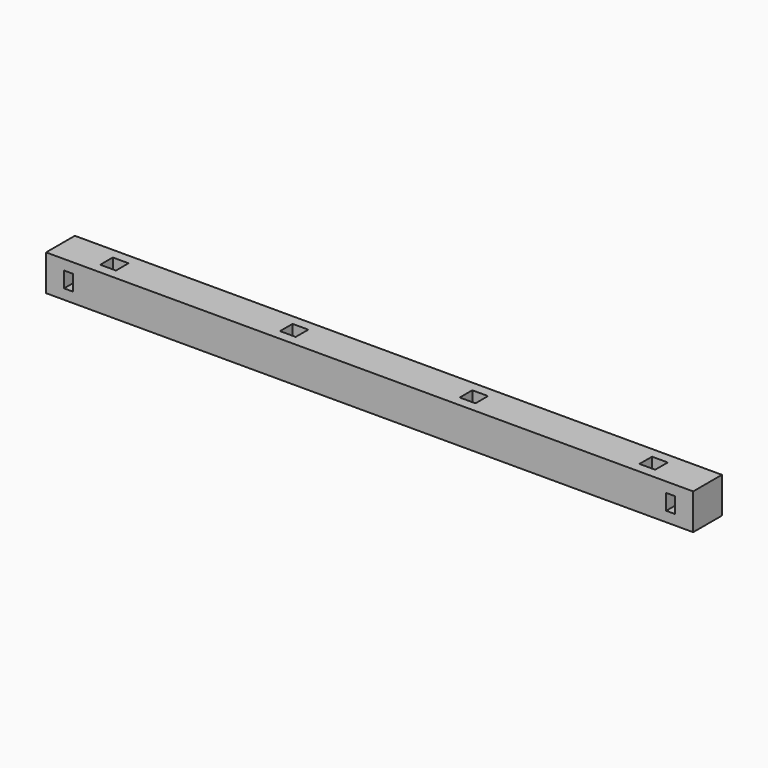
from build123d import *

# Parameters (mm, degrees)
F0_W            = 101.6
F0_H            = 101.6
F1_DEPTH        = 914.4
F2_W            = 44.45
F2_H            = 44.45
F3_DEPTH        = 101.601
F4_W            = 44.45
F4_H            = 44.45
F5_DEPTH        = 101.601
F5_COPIES_COUNT = 3
F5_COPIES_PITCH = 508
F6_W            = 25.4
F6_H            = 44.45
F7_DEPTH        = 101.601


# Not quite as in the source:
# - a pattern or mirror of a feature is missing from the dataset's text; its kind, count and spacing are read off the source's solid


with BuildPart() as f1:
    # F0 (on Right) → F1 (new body, symmetric)
    with BuildSketch(Plane.YZ):
        Rectangle(F0_W, F0_H)
    extrude(amount=F1_DEPTH, both=True)

    # F2 (on face) → F3 (cut, through all)
    with BuildSketch(Plane.XY.offset(50.8)):
        with Locations((-762, 0)):
            Rectangle(F2_W, F2_H)
    extrude(amount=-F3_DEPTH, mode=Mode.SUBTRACT)

    # F4 (on face) → F5 (cut, through all)
    with BuildSketch(Plane.XY.offset(50.8)):
        with Locations((-254, 0)):
            Rectangle(F4_W, F4_H)
    f5 = extrude(amount=-F5_DEPTH, mode=Mode.SUBTRACT)

    # F5_copies: F5 ×3
    with Locations(*[(i * F5_COPIES_PITCH, 0, 0) for i in range(1, F5_COPIES_COUNT)]):
        add(f5, mode=Mode.SUBTRACT)

    # F6 (on face) → F7 (cut, through all)
    with BuildSketch(Plane.XZ.offset(50.8)):
        with Locations((-850.9, 0)):
            Rectangle(F6_W, F6_H)
    f7 = extrude(amount=-F7_DEPTH, mode=Mode.SUBTRACT)

    # F7_copies: F7 across plane
    add(f7.mirror(Plane(origin=(0, 0, 0), x_dir=(0, 0, 1), z_dir=(1, 0, 0))), mode=Mode.SUBTRACT)


solid = f1.part
